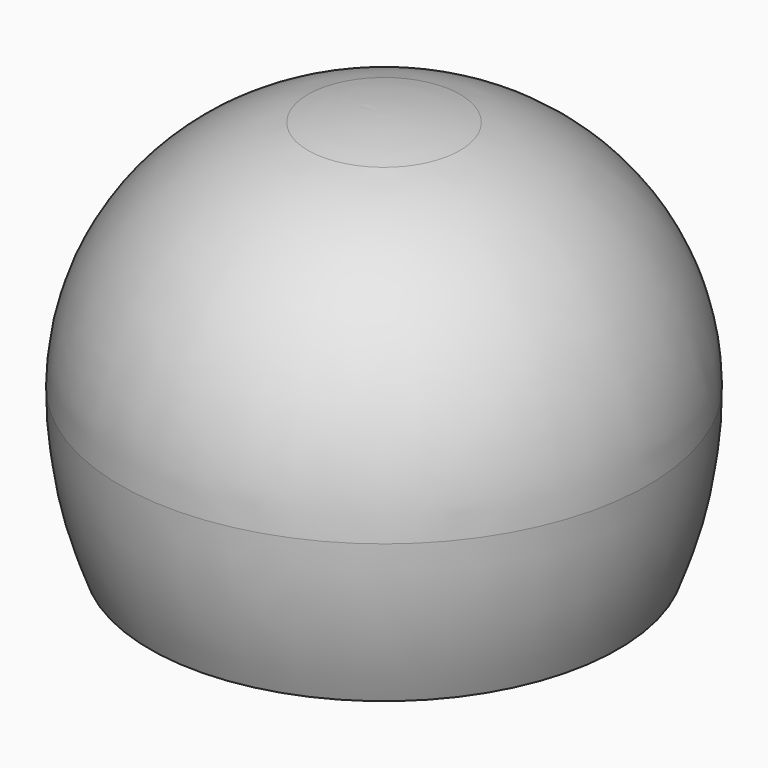
from build123d import *

# Parameters (mm, degrees)
F2_R = 1.2
F3_R = 1.5


# Not quite as in the source:
# - ends of sketch curves that miss each other by under 0.0002 mm in the source are joined


with BuildPart() as f1:
    # F0 (on Front) → F1 (revolve)
    with BuildSketch(Plane.XZ):
        with BuildLine():
            ThreePointArc((-4.2857142857, 22.0354204731), (-4.4681645184, 21.9940159633), (-4.65, 21.949990079))
            Line((-4.65, 21.949990079), (-4.65, 17.7503797432))
            Line((-4.65, 17.7503797432), (-3.15, 17.7503797432))
            Line((-3.15, 17.7503797432), (-3.15, 22.2503797432))
            ThreePointArc((-3.15, 22.2503797432), (-3.7194103843, 22.1511064929), (-4.2857142857, 22.0354204731))
        make_face()
        with BuildLine():
            ThreePointArc((-6.6773964801, 21.2619334538), (-5.6778868479, 21.6477692756), (-4.65, 21.949990079))
            ThreePointArc((-4.65, 21.949990079), (-4.4681645184, 21.9940159633), (-4.2857142857, 22.0354204731))
            ThreePointArc((-4.2857142857, 22.0354204731), (-3.7194103843, 22.1511064929), (-3.15, 22.2503797432))
            ThreePointArc((-3.15, 22.2503797432), (-1.5799375203, 22.437497271), (0, 22.5))
            Line((0, 22.5), (0, 24))
            ThreePointArc((0, 24), (-2.3170665414, 23.8747799947), (-4.6071429427, 23.5005773988))
            ThreePointArc((-4.6071429427, 23.5005773988), (-12.7983092871, 18.4257533886), (-16.0000003995, 9.3373971656))
            ThreePointArc((-16.0000003995, 9.3373971656), (-15.5435321148, 4.5818686667), (-14.1907963241, 0))
            Line((-14.1907963241, 0), (-12.5653197095, 0))
            ThreePointArc((-12.5653197095, 0), (-14.0112473931, 4.5695367006), (-14.5, 9.3373971656))
            ThreePointArc((-14.5, 9.3373971656), (-12.3698241532, 16.4680999977), (-6.6773964801, 21.2619334538))
        make_face()
        with BuildLine():
            Line((-4.65, 17.7503797432), (-4.65, 21.949990079))
            ThreePointArc((-4.65, 21.949990079), (-5.6778868479, 21.6477692756), (-6.6773964801, 21.2619334538))
            Line((-6.6773964801, 21.2619334538), (-4.65, 17.7503797432))
        make_face()
    revolve(axis=Axis((0, 0, 23.25), (0, 0, 1)))

    # F2
    f2_edges = [f1.edges().sort_by_distance(p)[0] for p in [
        (3.15, 0, 17.75038),
    ]]
    fillet(f2_edges, radius=F2_R)

    # F3
    f3_edges = [f1.edges().sort_by_distance(p)[0] for p in [
        (6.677396, 0, 21.261933),
    ]]
    fillet(f3_edges, radius=F3_R)


solid = f1.part
